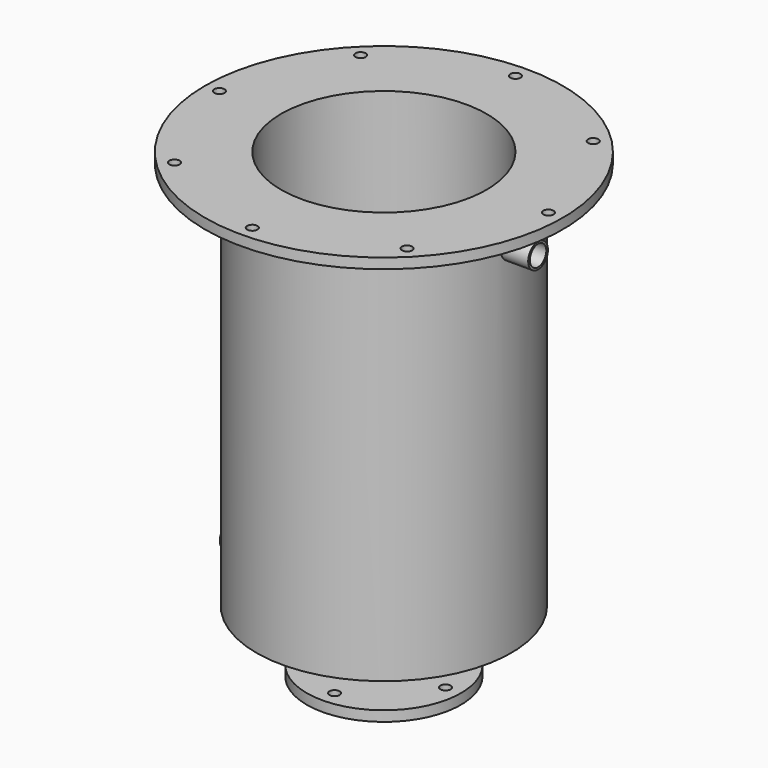
from build123d import *

# Parameters (mm, degrees)
F0_W          = 20
F0_H          = 376.8444419045
F6_END_RADIUS = 124
F5_R          = 12
F6_REACH      = 357.942125497
F4_R          = 10
F7_DEPTH      = 30
F9_R          = 12
F9_R_2        = 10
F11_R         = 10
F12_DEPTH     = 30
F13_R         = 5
F14_DEPTH     = 10
F15_R         = 5
F16_DEPTH     = 10


with BuildPart() as f1:
    # F0 (on Front) → F1 (revolve)
    with BuildSketch(Plane.XZ):
        with BuildLine():
            Line((-100, 12.7016653793), (-100, 400))
            Line((-100, 400), (-102, 400))
            Line((-102, 400), (-124, 400))
            Line((-124, 400), (-174, 400))
            Line((-174, 400), (-174, 390))
            Line((-174, 390), (-124, 390))
            Line((-124, 390), (-124, 11.1555580955))
            Line((-124, 11.1555580955), (-102, 11.1555580955))
            ThreePointArc((-102, 11.1555580955), (-64.7900629275, 3.2554376606), (-27, -1.0922587136))
            Line((-27, -1.0922587136), (-27, -39.2179855668))
            Line((-27, -39.2179855668), (-75, -39.2179855668))
            Line((-75, -39.2179855668), (-75, -49.2179855668))
            Line((-75, -49.2179855668), (-25, -49.2179855668))
            Line((-25, -49.2179855668), (-25, 0.7820144332))
            ThreePointArc((-25, 0.7820144332), (-62.7835131198, 4.9579383403), (-100, 12.7016653793))
        make_face()
        with Locations((-112, 201.5777790478)):
            Rectangle(F0_W, F0_H, mode=Mode.SUBTRACT)
    revolve(axis=Axis((0, 0, 200), (0, 0, 1)))

    f6_end = (Plane(origin=(0, 0, 200.5777790478), x_dir=(-1, 0, 0), z_dir=(0, 0, -1)) * Cylinder(F6_END_RADIUS, 2048.5579523277, mode=Mode.PRIVATE)).faces().sort_by_distance((124, 0, 200.5777790478))[0]
    # F5 (on offset) → F6 (join, up to the whole of a round face its end follows)
    with BuildSketch(Plane.YZ.offset(-150)):
        with Locations((0, 23)):
            Circle(F5_R)
    f6_long = extrude(amount=F6_REACH, mode=Mode.PRIVATE)
    add(split(f6_long, bisect_by=f6_end, keep=Keep.ALL, mode=Mode.PRIVATE).solids().sort_by_distance((-150, 0, 23))[0])

    # F4 (on offset) → F7 (cut)
    with BuildSketch(Plane.YZ.offset(-150)):
        with Locations((0, 23)):
            Circle(F4_R)
    extrude(amount=F7_DEPTH, mode=Mode.SUBTRACT)

    # F9 (on offset) → F10 (join, up to the next surface of F1)
    with BuildSketch(Plane.YZ.offset(150)):
        with Locations((0, 360)):
            Circle(F9_R)
        with Locations((0, 360)):
            Circle(F9_R_2, mode=Mode.SUBTRACT)
    extrude(until=Until.NEXT, dir=(-1, 0, 0))

    # F11 (on offset) → F12 (cut)
    with BuildSketch(Plane.YZ.offset(150)):
        with Locations((0, 360)):
            Circle(F11_R)
    extrude(amount=-F12_DEPTH, mode=Mode.SUBTRACT)

    # F13 (on face) → F14 (cut, through all)
    with BuildSketch(Plane(origin=(0, 0, -49.2179855668), x_dir=(1, 0, 0), z_dir=(0, 0, -1))):
        with Locations((0, 60)):
            Circle(F13_R)
        with Locations((60, 0)):
            Circle(F13_R)
        with Locations((0, -60)):
            Circle(F13_R)
        with Locations((-60, 0)):
            Circle(F13_R)
    extrude(amount=-F14_DEPTH, mode=Mode.SUBTRACT)

    # F15 (on face) → F16 (cut, through all)
    with BuildSketch(Plane.XY.offset(400)):
        with Locations((0, 160)):
            Circle(F15_R)
        with Locations((-113.1370849898, 113.1370849898)):
            Circle(F15_R)
        with Locations((-160, 0)):
            Circle(F15_R)
        with Locations((-113.1370849898, -113.1370849898)):
            Circle(F15_R)
        with Locations((0, -160)):
            Circle(F15_R)
        with Locations((113.1370849898, -113.1370849898)):
            Circle(F15_R)
        with Locations((160, 0)):
            Circle(F15_R)
        with Locations((113.1370849898, 113.1370849898)):
            Circle(F15_R)
    extrude(amount=-F16_DEPTH, mode=Mode.SUBTRACT)


solid = f1.part
